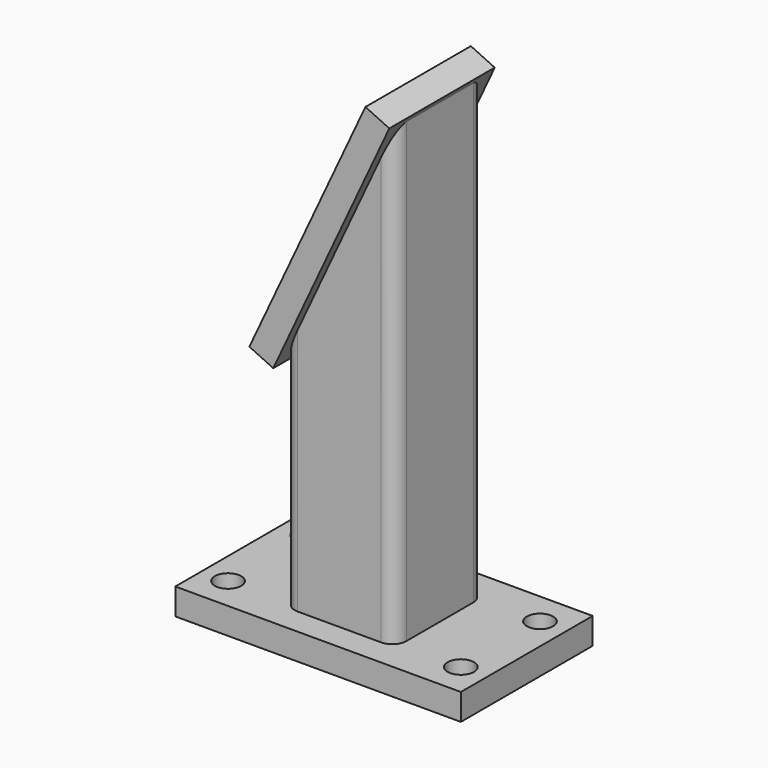
from build123d import *

# Parameters (mm, degrees)
F0_W     = 130
F0_H     = 75
F1_DEPTH = 12
F3_DEPTH = 208.083
F5_D     = 12
F7_DEPTH = 50.8
F8_W     = 60
F8_H     = 125
F9_DEPTH = 12


with BuildPart() as f1:
    # F0 (on Top) → F1 (new body)
    with BuildSketch(Plane.XY):
        Rectangle(F0_W, F0_H)
    extrude(amount=-F1_DEPTH)

    # F2 (on face) → F3 (join)
    with BuildSketch(Plane.XY):
        with BuildLine():
            Line((-19.05, -25.4), (19.05, -25.4))
            ThreePointArc((19.05, -25.4), (23.5401280605, -23.5401280605), (25.4, -19.05))
            Line((25.4, -19.05), (25.4, 19.05))
            ThreePointArc((25.4, 19.05), (23.5401280605, 23.5401280605), (19.05, 25.4))
            Line((19.05, 25.4), (-19.05, 25.4))
            ThreePointArc((-19.05, 25.4), (-23.5401280605, 23.5401280605), (-25.4, 19.05))
            Line((-25.4, 19.05), (-25.4, -19.05))
            ThreePointArc((-25.4, -19.05), (-23.5401280605, -23.5401280605), (-19.05, -25.4))
        make_face()
        with BuildLine():
            Line((-12.7, 19.05), (12.7, 19.05))
            ThreePointArc((12.7, 19.05), (17.1901280605, 17.1901280605), (19.05, 12.7))
            Line((19.05, 12.7), (19.05, -12.7))
            ThreePointArc((19.05, -12.7), (17.1901280605, -17.1901280605), (12.7, -19.05))
            Line((12.7, -19.05), (-12.7, -19.05))
            ThreePointArc((-12.7, -19.05), (-17.1901280605, -17.1901280605), (-19.05, -12.7))
            Line((-19.05, -12.7), (-19.05, 12.7))
            ThreePointArc((-19.05, 12.7), (-17.1901280605, 17.1901280605), (-12.7, 19.05))
        make_face(mode=Mode.SUBTRACT)
    extrude(amount=F3_DEPTH)

    # F5 (through all)
    with Locations(Plane.XY):
        with Locations((-53, 22.5), (53, 22.5), (53, -22.5), (-53, -22.5)):
            Hole(F5_D / 2)

    # F6 (on face) → F7 (cut)
    with BuildSketch(Plane.XZ.offset(25.4)):
        Polygon((19.05, 208.083), (-19.05, 208.083), (-19.05, 112.7596673834), (19.05, 194.4653810548), align=None)
        Polygon((25.4, 208.083), (19.05, 208.083), (19.05, 194.4653810548), align=None)
        Polygon((-19.05, 112.7596673834), (-19.05, 208.083), (-25.4, 208.083), (-25.4, 99.1420484381), align=None)
    extrude(amount=-F7_DEPTH, mode=Mode.SUBTRACT)

    # F8 (on face) → F9 (join)
    with BuildSketch(Plane(origin=(-58.8370102857, 0, 27.4361484792), x_dir=(0, -1, 0), z_dir=(-0.906307787, 0, 0.4226182617))):
        with Locations((0, 139.2202268861)):
            Rectangle(F8_W, F8_H)
        with BuildLine():
            Line((25.4, 184.2963670451), (25.4, 94.144086727))
            add(Edge.make_bspline(
                [(25.4, 94.144086727), (25.4, 79.118706674), (19.05, 79.118706674)],
                knots=[4.7123889804, 4.7123889804, 4.7123889804, 6.2831853072, 6.2831853072, 6.2831853072], degree=2, weights=[1, 0.7071067812, 1]))
            Line((19.05, 79.118706674), (-19.05, 79.118706674))
            add(Edge.make_bspline(
                [(-19.05, 79.118706674), (-25.4, 79.118706674), (-25.4, 94.144086727)],
                knots=[0, 0, 0, 1.5707963268, 1.5707963268, 1.5707963268], degree=2, weights=[1, 0.7071067812, 1]))
            Line((-25.4, 94.144086727), (-25.4, 184.2963670451))
            add(Edge.make_bspline(
                [(-25.4, 184.2963670451), (-25.4, 199.3217470982), (-19.05, 199.3217470982)],
                knots=[1.5707963268, 1.5707963268, 1.5707963268, 3.1415926536, 3.1415926536, 3.1415926536], degree=2, weights=[1, 0.7071067812, 1]))
            Line((-19.05, 199.3217470982), (19.05, 199.3217470982))
            add(Edge.make_bspline(
                [(19.05, 199.3217470982), (25.4, 199.3217470982), (25.4, 184.2963670451)],
                knots=[3.1415926536, 3.1415926536, 3.1415926536, 4.7123889804, 4.7123889804, 4.7123889804], degree=2, weights=[1, 0.7071067812, 1]))
        make_face(mode=Mode.SUBTRACT)
        with BuildLine():
            add(Edge.make_bspline(
                [(25.4, 94.144086727), (25.4, 79.118706674), (19.05, 79.118706674)],
                knots=[4.7123889804, 4.7123889804, 4.7123889804, 6.2831853072, 6.2831853072, 6.2831853072], degree=2, weights=[1, 0.7071067812, 1]))
            Line((25.4, 94.144086727), (25.4, 184.2963670451))
            add(Edge.make_bspline(
                [(19.05, 199.3217470982), (25.4, 199.3217470982), (25.4, 184.2963670451)],
                knots=[3.1415926536, 3.1415926536, 3.1415926536, 4.7123889804, 4.7123889804, 4.7123889804], degree=2, weights=[1, 0.7071067812, 1]))
            Line((19.05, 199.3217470982), (-19.05, 199.3217470982))
            add(Edge.make_bspline(
                [(-25.4, 184.2963670451), (-25.4, 199.3217470982), (-19.05, 199.3217470982)],
                knots=[1.5707963268, 1.5707963268, 1.5707963268, 3.1415926536, 3.1415926536, 3.1415926536], degree=2, weights=[1, 0.7071067812, 1]))
            Line((-25.4, 184.2963670451), (-25.4, 94.144086727))
            add(Edge.make_bspline(
                [(-19.05, 79.118706674), (-25.4, 79.118706674), (-25.4, 94.144086727)],
                knots=[0, 0, 0, 1.5707963268, 1.5707963268, 1.5707963268], degree=2, weights=[1, 0.7071067812, 1]))
            Line((-19.05, 79.118706674), (19.05, 79.118706674))
        make_face()
        with BuildLine():
            Line((12.7, 94.144086727), (-12.7, 94.144086727))
            add(Edge.make_bspline(
                [(-12.7, 94.144086727), (-19.05, 94.144086727), (-19.05, 109.1694667801)],
                knots=[0, 0, 0, 1.5707963268, 1.5707963268, 1.5707963268], degree=2, weights=[1, 0.7071067812, 1]))
            Line((-19.05, 109.1694667801), (-19.05, 169.2709869921))
            add(Edge.make_bspline(
                [(-19.05, 169.2709869921), (-19.05, 184.2963670451), (-12.7, 184.2963670451)],
                knots=[1.5707963268, 1.5707963268, 1.5707963268, 3.1415926536, 3.1415926536, 3.1415926536], degree=2, weights=[1, 0.7071067812, 1]))
            Line((-12.7, 184.2963670451), (12.7, 184.2963670451))
            add(Edge.make_bspline(
                [(12.7, 184.2963670451), (19.05, 184.2963670451), (19.05, 169.2709869921)],
                knots=[3.1415926536, 3.1415926536, 3.1415926536, 4.7123889804, 4.7123889804, 4.7123889804], degree=2, weights=[1, 0.7071067812, 1]))
            Line((19.05, 169.2709869921), (19.05, 109.1694667801))
            add(Edge.make_bspline(
                [(19.05, 109.1694667801), (19.05, 94.144086727), (12.7, 94.144086727)],
                knots=[4.7123889804, 4.7123889804, 4.7123889804, 6.2831853072, 6.2831853072, 6.2831853072], degree=2, weights=[1, 0.7071067812, 1]))
        make_face(mode=Mode.SUBTRACT)
        with BuildLine():
            add(Edge.make_bspline(
                [(-12.7, 94.144086727), (-19.05, 94.144086727), (-19.05, 109.1694667801)],
                knots=[0, 0, 0, 1.5707963268, 1.5707963268, 1.5707963268], degree=2, weights=[1, 0.7071067812, 1]))
            Line((-12.7, 94.144086727), (12.7, 94.144086727))
            add(Edge.make_bspline(
                [(19.05, 109.1694667801), (19.05, 94.144086727), (12.7, 94.144086727)],
                knots=[4.7123889804, 4.7123889804, 4.7123889804, 6.2831853072, 6.2831853072, 6.2831853072], degree=2, weights=[1, 0.7071067812, 1]))
            Line((19.05, 109.1694667801), (19.05, 169.2709869921))
            add(Edge.make_bspline(
                [(12.7, 184.2963670451), (19.05, 184.2963670451), (19.05, 169.2709869921)],
                knots=[3.1415926536, 3.1415926536, 3.1415926536, 4.7123889804, 4.7123889804, 4.7123889804], degree=2, weights=[1, 0.7071067812, 1]))
            Line((12.7, 184.2963670451), (-12.7, 184.2963670451))
            add(Edge.make_bspline(
                [(-19.05, 169.2709869921), (-19.05, 184.2963670451), (-12.7, 184.2963670451)],
                knots=[1.5707963268, 1.5707963268, 1.5707963268, 3.1415926536, 3.1415926536, 3.1415926536], degree=2, weights=[1, 0.7071067812, 1]))
            Line((-19.05, 169.2709869921), (-19.05, 109.1694667801))
        make_face()
    extrude(amount=F9_DEPTH)


solid = f1.part
